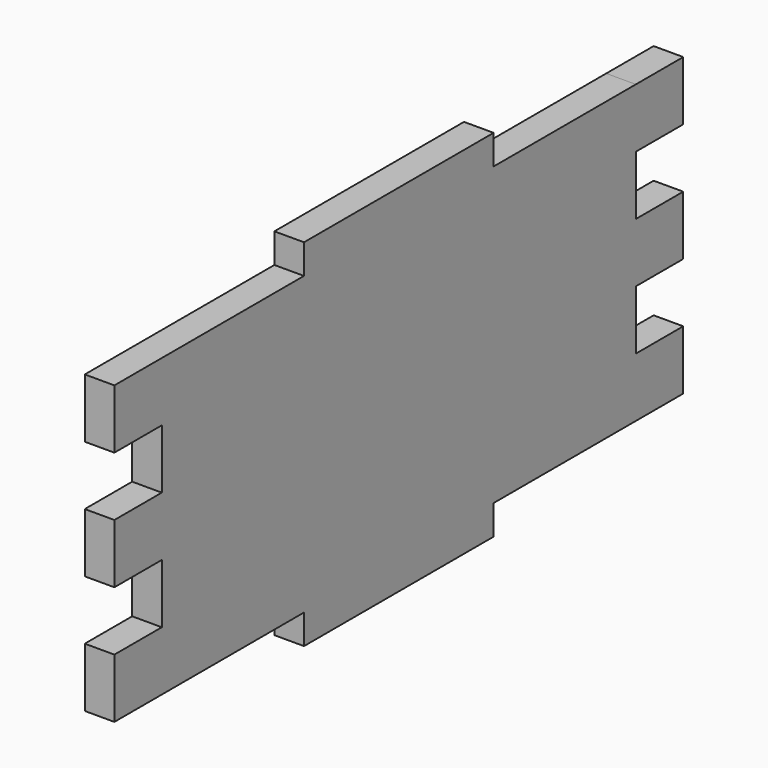
from build123d import *

# Parameters (mm, degrees)
F0_W     = 12.7
F0_H     = 12.7
F0_W_2   = 50.8
F0_H_2   = 6.35
F1_DEPTH = 6.35


# Not quite as in the source:
# - ends of sketch curves that miss each other by under 0.0002 mm in the source are joined


with BuildPart() as f1:
    # F0 (on Right) → F1 (new body)
    with BuildSketch(Plane.YZ):
        with Locations((-31.75, 6.35)):
            Rectangle(F0_W, F0_H)
        Polygon((12.7, 12.7), (-25.4, 12.7), (-25.4, 0), (-25.4, -12.7), (-25.4, -25.4), (-25.4, -38.1), (-25.4, -50.8), (12.7, -50.8), (63.5, -50.8), (101.6, -50.8), (101.6, -38.0999993861), (101.6, -25.3999993861), (101.6, -12.6999993861), (101.6, 6.139e-07), (101.6, 12.7), (63.5, 12.7), align=None)
        with Locations((-31.75, -19.05)):
            Rectangle(F0_W, F0_H)
        with Locations((-31.75, -44.45)):
            Rectangle(F0_W, F0_H)
        with Locations((38.1, -53.975)):
            Rectangle(F0_W_2, F0_H_2)
        with Locations((38.1, 15.875)):
            Rectangle(F0_W_2, F0_H_2)
        with Locations((107.95, 6.3500006139)):
            Rectangle(F0_W, F0_H)
        with Locations((107.95, -19.0499993861)):
            Rectangle(F0_W, F0_H)
        Polygon((114.3, -38.0999993861), (101.6, -38.0999993861), (101.6, -50.8), (114.3, -50.7999993861), align=None)
    extrude(amount=F1_DEPTH)


solid = f1.part
